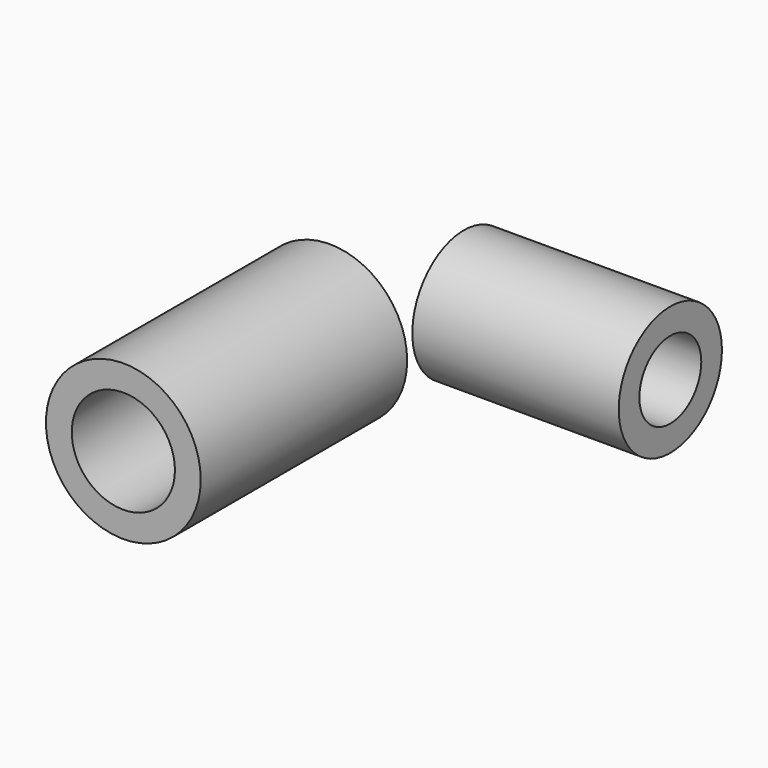
from build123d import *

# Parameters (mm, degrees)
F0_R     = 19.05
F0_R_2   = 12.7
F2_DEPTH = 63.5
F3_R     = 15.875
F3_R_2   = 9.525
F5_DEPTH = 50.8


# Not quite as in the source:
# - a variable given as a bare number and used for a length is read in inches; the dataset says mm whatever the document's units were


with BuildPart() as f2:
    # F0 (on Front) → F2 (new body)
    with BuildSketch(Plane.XZ):
        with Locations((-63.5, 0)):
            Circle(F0_R)
        with Locations((-63.5, 0)):
            Circle(F0_R_2, mode=Mode.SUBTRACT)
    extrude(amount=-F2_DEPTH)


with BuildPart() as f5:
    # F3 (on Right) → F5 (new body)
    with BuildSketch(Plane.YZ):
        with Locations((88.9, 0)):
            Circle(F3_R)
        with Locations((88.9, 0)):
            Circle(F3_R_2, mode=Mode.SUBTRACT)
    extrude(amount=-F5_DEPTH)


solid = Compound([f2.part, f5.part])
